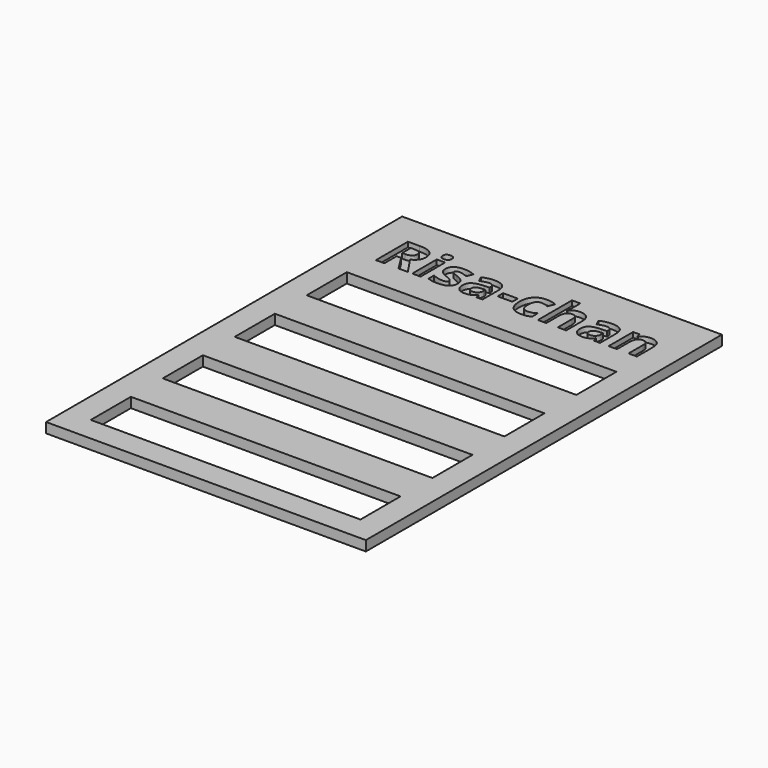
from build123d import *

# Parameters (mm, degrees)
F0_W         = 63.8
F0_H         = 88.8
F1_DEPTH     = 2
F2_TEXT_SIZE = 11.1839412739
F3_DEPTH     = 1
F4_W         = 53.8
F4_H         = 10
F5_DEPTH     = 25


# Not quite as in the source:
# - Text() gives the source's letters only with a copy of the font that has no kerning and outlines rounded to 1/6400 em; it was checked with that copy


with BuildPart() as f1:
    # F0 (on Top) → F1 (new body)
    with BuildSketch(Plane.XY):
        Rectangle(F0_W, F0_H)
    extrude(amount=F1_DEPTH)

    # F2 (on face) → F3 (cut)
    with BuildSketch(Plane.XY.offset(2)):
        with Locations((-26.9, 30.3475622828)):
            Text('Risa-chan', F2_TEXT_SIZE, font='Open Sans', font_style=FontStyle.BOLD, text_align=(TextAlign.LEFT, TextAlign.BOTTOM))
    extrude(amount=-F3_DEPTH, mode=Mode.SUBTRACT)

    # F4 (on face) → F5 (cut)
    with BuildSketch(Plane.XY.offset(2)):
        with Locations((0, 19.3475622828)):
            Rectangle(F4_W, F4_H)
        with Locations((0, 1.3983748552)):
            Rectangle(F4_W, F4_H)
        with Locations((0, -16.5508125724)):
            Rectangle(F4_W, F4_H)
        with Locations((0, -34.5)):
            Rectangle(F4_W, F4_H)
    extrude(amount=-F5_DEPTH, mode=Mode.SUBTRACT)


solid = f1.part
